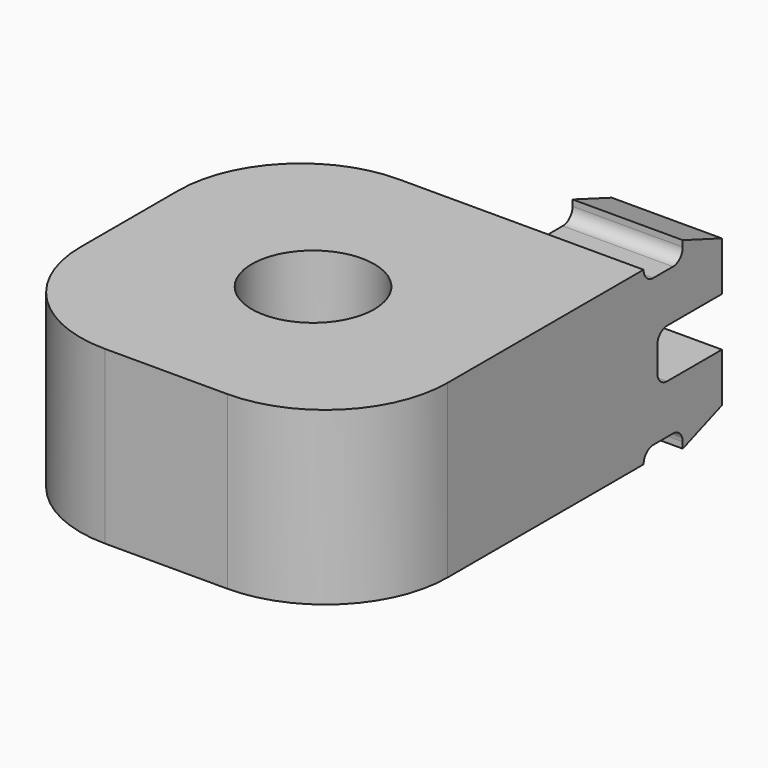
from build123d import *

# Parameters (mm, degrees)
F0_W        = 15
F0_H        = 15
F0_R        = 2.5
F1_DEPTH    = 7
F2_W        = 0.7
F2_H        = 2
F3_DEPTH    = 4.5
F4_T1_DEPTH = 4.5
F5_R        = 5


# Not quite as in the source:
# - a fillet or chamfer that OpenCascade refuses, or shapes differently, is made with other operations: its cross-section is extruded or revolved along the edge and cut away or added


with BuildPart() as f1:
    # F0 (on Top) → F1 (new body)
    with BuildSketch(Plane.XY):
        with Locations((-9.923633188, 7.5)):
            Rectangle(F0_W, F0_H)
        with Locations((-9.923633188, 7.5)):
            Circle(F0_R, mode=Mode.SUBTRACT)
    extrude(amount=F1_DEPTH)

    # F2 (on face) → F3 (join)
    with BuildSketch(Plane.YZ.offset(-2.423633188)):
        Polygon((17, 7.25), (17, 6.5), (19, 6.5), align=None)
        Polygon((17, 6.5), (15, 6.5), (15, 4.5), (15.7, 4.5), (19, 4.5), (19, 6.5), align=None)
        with Locations((15.35, 3.5)):
            Rectangle(F2_W, F2_H)
        Polygon((15.7, 2.5), (15, 2.5), (15, 0.5), (17, 0.5), (19, 0.5), (19, 2.5), align=None)
        Polygon((19, 0.5), (17, 0.5), (17, -0.25), align=None)
    extrude(amount=-F3_DEPTH)

    # F4: fillet of radius 0.5 on 7 edges, made by hand

    # F4_s2 → F4_t1 (join)
    with BuildSketch(Plane.YZ.offset(-6.923633188)):
        with BuildLine():
            ThreePointArc((16.2, 2.5), (15.8464466094, 2.6464466094), (15.7, 3))
            Line((15.7, 3), (15.7, 2.5))
            Line((15.7, 2.5), (16.2, 2.5))
        make_face()
        with BuildLine():
            ThreePointArc((15.7, 4), (15.8464466094, 4.3535533906), (16.2, 4.5))
            Line((16.2, 4.5), (15.7, 4.5))
            Line((15.7, 4.5), (15.7, 4))
        make_face()
        with BuildLine():
            ThreePointArc((16.5, 0.5), (16.8535533906, 0.3535533906), (17, 0))
            Line((17, 0), (17, 0.5))
            Line((17, 0.5), (16.5, 0.5))
        make_face()
        with BuildLine():
            ThreePointArc((16.5, 6.5), (16.8535533906, 6.6464466094), (17, 7))
            Line((17, 7), (17, 6.5))
            Line((17, 6.5), (16.5, 6.5))
        make_face()
        with BuildLine():
            ThreePointArc((15, 7), (15.1464466094, 6.6464466094), (15.5, 6.5))
            Line((15.5, 6.5), (15, 6.5))
            Line((15, 6.5), (15, 7))
        make_face()
        with BuildLine():
            ThreePointArc((15, 0), (15.1464466094, 0.3535533906), (15.5, 0.5))
            Line((15.5, 0.5), (15, 0.5))
            Line((15, 0.5), (15, 0))
        make_face()
    extrude(amount=F4_T1_DEPTH)

    # F5
    f5_edges = [f1.edges().sort_by_distance(p)[0] for p in [
        (-17.423633, 15, 3.5),
        (-17.423633, 0, 3.5),
        (-2.423633, 0, 3.5),
    ]]
    fillet(f5_edges, radius=F5_R)


solid = f1.part
